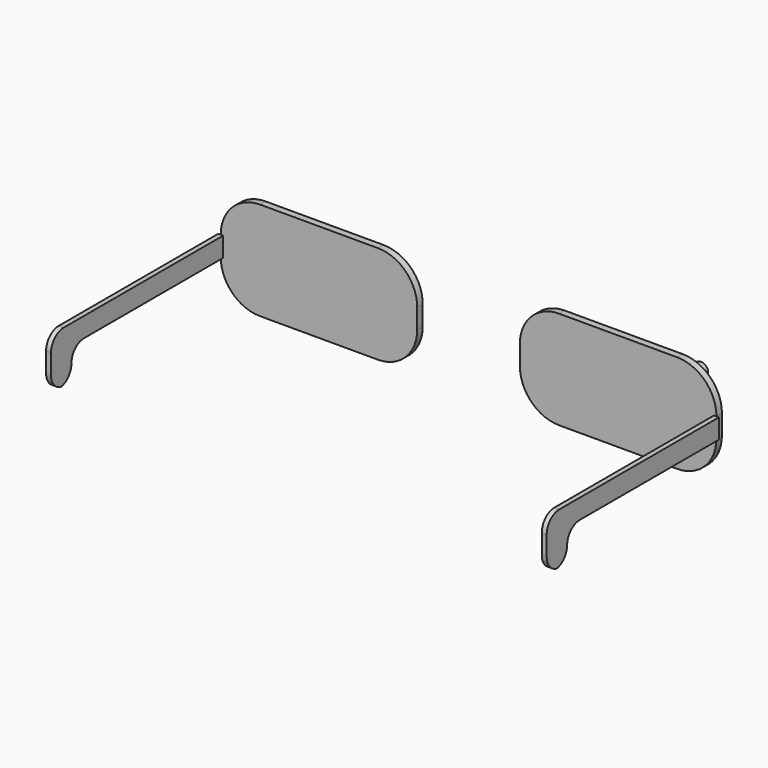
from build123d import *

# Parameters (mm, degrees)
F0_W        = 25.4
F0_H        = 12.7
F1_DEPTH    = 0.889
F2_R        = 5.08
F2_2_R      = 5.08
F5_DEPTH    = 0.3175
F6_T1_DEPTH = 0.635
F6_T3_DEPTH = 10.795
F8_DEPTH    = 0.3175
F9_T1_DEPTH = 0.635
F9_T3_DEPTH = 10.795
F10_R       = 0.9381315748
F10_R_2     = 0.643552657
F10_R_3     = 0.4022191612
F11_DEPTH   = 0.6858


# Not quite as in the source:
# - a fillet or chamfer that OpenCascade refuses, or shapes differently, is made with other operations: its cross-section is extruded or revolved along the edge and cut away or added
# - a feature names something its author has since deleted; it is built from what else it names
# - the program builds the solid bodies; features that only make, move or delete a surface that nothing else refers to are left out


with BuildPart() as f1:
    # F0 (on Front) → F1 (new body)
    with BuildSketch(Plane.XZ):
        with Locations((-25.9656485498, 29.3908948079)):
            Rectangle(F0_W, F0_H)
    extrude(amount=F1_DEPTH)

    # F2
    f2_edges = [f1.edges().sort_by_distance(p)[0] for p in [
        (-38.665649, -0.4445, 35.740895),
        (-38.665649, -0.4445, 23.040895),
        (-13.265649, -0.4445, 23.040895),
        (-13.265649, -0.4445, 35.740895),
    ]]
    fillet(f2_edges, radius=F2_R)


with BuildPart() as f1b:
    # F0 (on Front) → F1, piece 2 (new body)
    with BuildSketch(Plane.XZ):
        with Locations((12.7, 29.546997121)):
            Rectangle(F0_W, F0_H)
    extrude(amount=F1_DEPTH)

    # F2#2
    f2_2_edges = [f1b.edges().sort_by_distance(p)[0] for p in [
        (0, -0.4445, 35.896997),
        (0, -0.4445, 23.196997),
        (25.4, -0.4445, 23.196997),
        (25.4, -0.4445, 35.896997),
    ]]
    fillet(f2_2_edges, radius=F2_2_R)

    # F10 (on face) → F11 (join)
    with BuildSketch(Plane(origin=(0, 0, 0), x_dir=(-1, 0, 0), z_dir=(0, 1, 0))):
        with Locations((-22.1409089863, 34.4025939703)):
            Circle(F10_R)
        with Locations((-22.1409089863, 34.4025939703)):
            Circle(F10_R_2, mode=Mode.SUBTRACT)
        with Locations((-22.1409089863, 34.4025939703)):
            Circle(F10_R_2)
        with Locations((-22.1409089863, 34.4025939703)):
            Circle(F10_R_3, mode=Mode.SUBTRACT)
        with Locations((-22.1409089863, 34.4025939703)):
            Circle(F10_R_3)
    extrude(amount=F11_DEPTH)


with BuildPart() as f5:
    # F4 (on face) → F5 (new body, symmetric)
    with BuildSketch(Plane.YZ.offset(25.4)):
        Polygon((-0.889, 28.276997121), (-0.889, 30.816997121), (-25.4, 30.816997121), (-28.702, 30.816997121), (-28.702, 24.212997121), (-25.4, 24.212997121), (-25.4, 28.276997121), align=None)
    extrude(amount=F5_DEPTH, both=True)

    # F6: fillet of radius 2.032 on 4 edges, made by hand

    # F6_s2 → F6_t1 (join)
    with BuildSketch(Plane.YZ.offset(25.0825)):
        with BuildLine():
            ThreePointArc((-23.368, 28.276997121), (-24.8048409794, 27.6818381003), (-25.4, 26.244997121))
            Line((-25.4, 26.244997121), (-25.4, 28.276997121))
            Line((-25.4, 28.276997121), (-23.368, 28.276997121))
        make_face()
    extrude(amount=F6_T1_DEPTH)

    # F6_s4 → F6_t3 (cut)
    with BuildSketch(Plane.YZ.offset(20.0025)):
        with BuildLine():
            ThreePointArc((-26.67, 30.816997121), (-28.1068409794, 30.2218381003), (-28.702, 28.784997121))
            Line((-28.702, 28.784997121), (-28.702, 30.816997121))
            Line((-28.702, 30.816997121), (-26.67, 30.816997121))
        make_face()
        with BuildLine():
            ThreePointArc((-28.702, 26.244997121), (-28.1068409794, 24.8081561416), (-26.67, 24.212997121))
            Line((-26.67, 24.212997121), (-28.702, 24.212997121))
            Line((-28.702, 24.212997121), (-28.702, 26.244997121))
        make_face()
        with BuildLine():
            ThreePointArc((-27.432, 24.212997121), (-25.9951590206, 24.8081561416), (-25.4, 26.244997121))
            Line((-25.4, 26.244997121), (-25.4, 24.212997121))
            Line((-25.4, 24.212997121), (-27.432, 24.212997121))
        make_face()
    extrude(amount=F6_T3_DEPTH, mode=Mode.SUBTRACT)


with BuildPart() as f8:
    # F7 (on face) → F8 (new body, symmetric)
    with BuildSketch(Plane(origin=(-38.6656485498, 0, 0), x_dir=(0, -1, 0), z_dir=(-1, 0, 0))):
        Polygon((25.4, 30.6608948079), (0.889, 30.6608948079), (0.889, 28.1208948079), (25.4, 28.1208948079), (25.4, 24.0568948079), (28.702, 24.0568948079), (28.702, 30.6608948079), align=None)
    extrude(amount=F8_DEPTH, both=True)

    # F9: fillet of radius 2.032 on 4 edges, made by hand

    # F9_s2 → F9_t1 (join)
    with BuildSketch(Plane.YZ.offset(-38.9831485498)):
        with BuildLine():
            ThreePointArc((-25.4, 26.0888948079), (-24.8048409794, 27.5257357872), (-23.368, 28.1208948079))
            Line((-23.368, 28.1208948079), (-25.4, 28.1208948079))
            Line((-25.4, 28.1208948079), (-25.4, 26.0888948079))
        make_face()
    extrude(amount=F9_T1_DEPTH)

    # F9_s4 → F9_t3 (cut)
    with BuildSketch(Plane.YZ.offset(-44.0631485498)):
        with BuildLine():
            ThreePointArc((-27.432, 24.0568948079), (-25.9951590206, 24.6520538285), (-25.4, 26.0888948079))
            Line((-25.4, 26.0888948079), (-25.4, 24.0568948079))
            Line((-25.4, 24.0568948079), (-27.432, 24.0568948079))
        make_face()
        with BuildLine():
            ThreePointArc((-26.67, 24.0568948079), (-28.1068409794, 24.6520538285), (-28.702, 26.0888948079))
            Line((-28.702, 26.0888948079), (-28.702, 24.0568948079))
            Line((-28.702, 24.0568948079), (-26.67, 24.0568948079))
        make_face()
        with BuildLine():
            ThreePointArc((-28.702, 28.6288948079), (-28.1068409794, 30.0657357872), (-26.67, 30.6608948079))
            Line((-26.67, 30.6608948079), (-28.702, 30.6608948079))
            Line((-28.702, 30.6608948079), (-28.702, 28.6288948079))
        make_face()
    extrude(amount=F9_T3_DEPTH, mode=Mode.SUBTRACT)


solid = Compound([f1.part, f1b.part, f5.part, f8.part])
